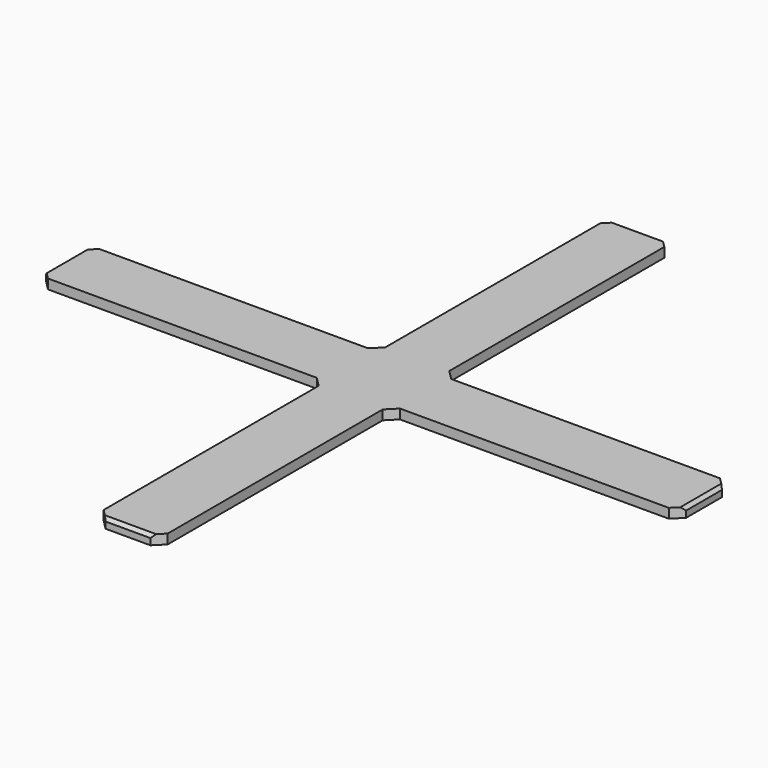
from build123d import *

# Parameters (mm, degrees)
F0_W     = 900
F0_H     = 200
F0_W_2   = 200
F0_H_2   = 900
F1_DEPTH = 30
F2_SIZE  = 30
F3_SIZE  = 10


with BuildPart() as f1:
    # F0 (on Top) → F1 (new body)
    with BuildSketch(Plane.XY):
        with Locations((-1543.7867450795, 647.8599071422)):
            Rectangle(F0_W, F0_H)
        with Locations((-993.7867450795, 1197.8599071422)):
            Rectangle(F0_W_2, F0_H_2)
        with Locations((-993.7867450795, 647.8599071422)):
            Rectangle(F0_W_2, F0_H)
        with Locations((-443.7867450795, 647.8599071422)):
            Rectangle(F0_W, F0_H)
        with Locations((-993.7867450795, 97.8599071422)):
            Rectangle(F0_W_2, F0_H_2)
    extrude(amount=F1_DEPTH)

    # F2
    f2_edges = [f1.edges().sort_by_distance(p)[0] for p in [
        (-1093.786745, 747.859907, 15),
        (-1993.786745, 747.859907, 15),
        (-1993.786745, 547.859907, 15),
        (-1093.786745, 547.859907, 15),
        (-1093.786745, -352.140093, 15),
        (-893.786745, -352.140093, 15),
        (-893.786745, 547.859907, 15),
        (6.213255, 547.859907, 15),
        (6.213255, 747.859907, 15),
        (-893.786745, 747.859907, 15),
        (-893.786745, 1647.859907, 15),
        (-1093.786745, 1647.859907, 15),
    ]]
    chamfer(f2_edges, length=F2_SIZE)

    # F3
    f3_edges = [f1.edges().sort_by_distance(p)[0] for p in [
        (-993.786745, -352.140093, 30),
        (6.213255, 647.859907, 30),
        (-993.786745, 1647.859907, 30),
        (-1993.786745, 647.859907, 30),
    ]]
    chamfer(f3_edges, length=F3_SIZE)


solid = f1.part
